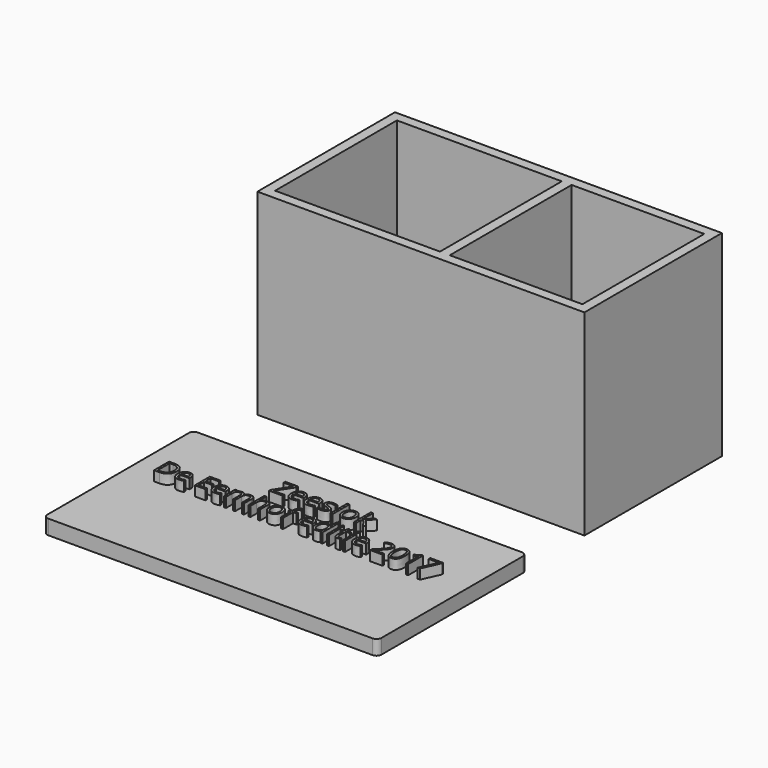
from build123d import *

# Parameters (mm, degrees)
F1_W           = 66.572660327
F1_H           = 35
F1_W_2         = 33.5726604834
F1_H_2         = 31
F1_W_3         = 26.9999998435
F2_DEPTH       = 40
F3_DEPTH       = 2
F4_DEPTH       = 2
F6_DEPTH       = 5
F7_DEPTH       = 3
F8_TEXT_SIZE   = 5.6227048238
F8_TEXT_SIZE_2 = 5.3549599316
F9_DEPTH       = 2


# Not quite as in the source:
# - Text() gives the source's letters only with a copy of the font that has no kerning and outlines rounded to 1/6400 em; it was checked with that copy


with BuildPart() as f2:
    # F1 (on Top) → F2 (new body)
    with BuildSketch(Plane.XY):
        with Locations((-12.7013317645, 0.3292801976)):
            Rectangle(F1_W, F1_H)
        with Locations((-27.2013316862, 0.3292801976)):
            Rectangle(F1_W_2, F1_H_2, mode=Mode.SUBTRACT)
        with Locations((5.0849984773, 0.3292801976)):
            Rectangle(F1_W_3, F1_H_2, mode=Mode.SUBTRACT)
    extrude(amount=F2_DEPTH)

    # F1 (on Top) → F3 (join)
    with BuildSketch(Plane.XY):
        with Locations((5.0849984773, 0.3292801976)):
            Rectangle(F1_W_3, F1_H_2)
    extrude(amount=F3_DEPTH)

    # F1 (on Top) → F4 (join)
    with BuildSketch(Plane.XY):
        with Locations((-27.2013316862, 0.3292801976)):
            Rectangle(F1_W_2, F1_H_2)
    extrude(amount=F4_DEPTH)


with BuildPart() as f6:
    # F5 (on Top) → F6 (new body)
    with BuildSketch(Plane.XY):
        with BuildLine():
            ThreePointArc((-10.0929591358, -31.8514965475), (-11.5071726981, -32.4372829851), (-12.0929591358, -33.8514965475))
            Line((-12.0929591358, -33.8514965475), (-12.0929591358, -59.8514965475))
            ThreePointArc((-12.0929591358, -59.8514965475), (-11.5071726981, -61.2657101098), (-10.0929591358, -61.8514965475))
            Line((-10.0929591358, -61.8514965475), (11.9070408642, -61.8514965475))
            ThreePointArc((11.9070408642, -61.8514965475), (13.3212544266, -61.2657101098), (13.9070408642, -59.8514965475))
            Line((13.9070408642, -59.8514965475), (13.9070408642, -33.8514965475))
            ThreePointArc((13.9070408642, -33.8514965475), (13.3212544266, -32.4372829851), (11.9070408642, -31.8514965475))
            Line((11.9070408642, -31.8514965475), (-10.0929591358, -31.8514965475))
        make_face()
    extrude(amount=-F6_DEPTH)



with BuildPart() as f6b:
    # F5 (on Top) → F6, piece 2 (new body)
    with BuildSketch(Plane.XY):
        with BuildLine():
            Line((-16.5929592848, -31.8514965475), (-45.0929592848, -31.8514965475))
            ThreePointArc((-45.0929592848, -31.8514965475), (-46.5071728472, -32.4372829851), (-47.0929592848, -33.8514965475))
            Line((-47.0929592848, -33.8514965475), (-47.0929592848, -59.8514965475))
            ThreePointArc((-47.0929592848, -59.8514965475), (-46.5071728472, -61.2657101098), (-45.0929592848, -61.8514965475))
            Line((-45.0929592848, -61.8514965475), (-16.5929592848, -61.8514965475))
            ThreePointArc((-16.5929592848, -61.8514965475), (-15.1787457224, -61.2657101098), (-14.5929592848, -59.8514965475))
            Line((-14.5929592848, -59.8514965475), (-14.5929592848, -33.8514965475))
            ThreePointArc((-14.5929592848, -33.8514965475), (-15.1787457224, -32.4372829851), (-16.5929592848, -31.8514965475))
        make_face()
    extrude(amount=-F6_DEPTH)


with BuildPart() as f6_1:
    add(f6.part)

    add(f6b.part)  # F7 merges F6b
    # F5 (on Top) → F7 (join)
    with BuildSketch(Plane.XY):
        with BuildLine():
            ThreePointArc((-49.5929592848, -27.8514965475), (-50.300066066, -28.1443897663), (-50.5929592848, -28.8514965475))
            Line((-50.5929592848, -28.8514965475), (-50.5929592848, -64.8514965475))
            ThreePointArc((-50.5929592848, -64.8514965475), (-50.300066066, -65.5586033286), (-49.5929592848, -65.8514965475))
            Line((-49.5929592848, -65.8514965475), (16.4070408642, -65.8514965475))
            ThreePointArc((16.4070408642, -65.8514965475), (17.1141476454, -65.5586033286), (17.4070408642, -64.8514965475))
            Line((17.4070408642, -64.8514965475), (17.4070408642, -28.8514965475))
            ThreePointArc((17.4070408642, -28.8514965475), (17.1141476454, -28.1443897663), (16.4070408642, -27.8514965475))
            Line((16.4070408642, -27.8514965475), (-49.5929592848, -27.8514965475))
        make_face()
        with BuildLine():
            ThreePointArc((-47.0929592848, -33.8514965475), (-46.5071728472, -32.4372829851), (-45.0929592848, -31.8514965475))
            Line((-45.0929592848, -31.8514965475), (-16.5929592848, -31.8514965475))
            ThreePointArc((-16.5929592848, -31.8514965475), (-15.1787457224, -32.4372829851), (-14.5929592848, -33.8514965475))
            Line((-14.5929592848, -33.8514965475), (-14.5929592848, -59.8514965475))
            ThreePointArc((-14.5929592848, -59.8514965475), (-15.1787457224, -61.2657101098), (-16.5929592848, -61.8514965475))
            Line((-16.5929592848, -61.8514965475), (-45.0929592848, -61.8514965475))
            ThreePointArc((-45.0929592848, -61.8514965475), (-46.5071728472, -61.2657101098), (-47.0929592848, -59.8514965475))
            Line((-47.0929592848, -59.8514965475), (-47.0929592848, -33.8514965475))
        make_face(mode=Mode.SUBTRACT)
        with BuildLine():
            Line((-12.0929591358, -59.8514965475), (-12.0929591358, -33.8514965475))
            ThreePointArc((-12.0929591358, -33.8514965475), (-11.5071726981, -32.4372829851), (-10.0929591358, -31.8514965475))
            Line((-10.0929591358, -31.8514965475), (11.9070408642, -31.8514965475))
            ThreePointArc((11.9070408642, -31.8514965475), (13.3212544266, -32.4372829851), (13.9070408642, -33.8514965475))
            Line((13.9070408642, -33.8514965475), (13.9070408642, -59.8514965475))
            ThreePointArc((13.9070408642, -59.8514965475), (13.3212544266, -61.2657101098), (11.9070408642, -61.8514965475))
            Line((11.9070408642, -61.8514965475), (-10.0929591358, -61.8514965475))
            ThreePointArc((-10.0929591358, -61.8514965475), (-11.5071726981, -61.2657101098), (-12.0929591358, -59.8514965475))
        make_face(mode=Mode.SUBTRACT)
    extrude(amount=-F7_DEPTH)

    # F8 (on Top) → F9 (join)
    with BuildSketch(Plane.XY):
        with Locations((-26.0250959545, -39.4231975079)):
            Text('Zeeslok', F8_TEXT_SIZE, font='Open Sans', text_align=(TextAlign.LEFT, TextAlign.BOTTOM))
        with Locations((-45.0137704611, -45.3511364758)):
            Text('De Eemhof editie 2017', F8_TEXT_SIZE_2, font='Open Sans', text_align=(TextAlign.LEFT, TextAlign.BOTTOM))
    extrude(amount=F9_DEPTH)


solid = Compound([f2.part, f6_1.part])
